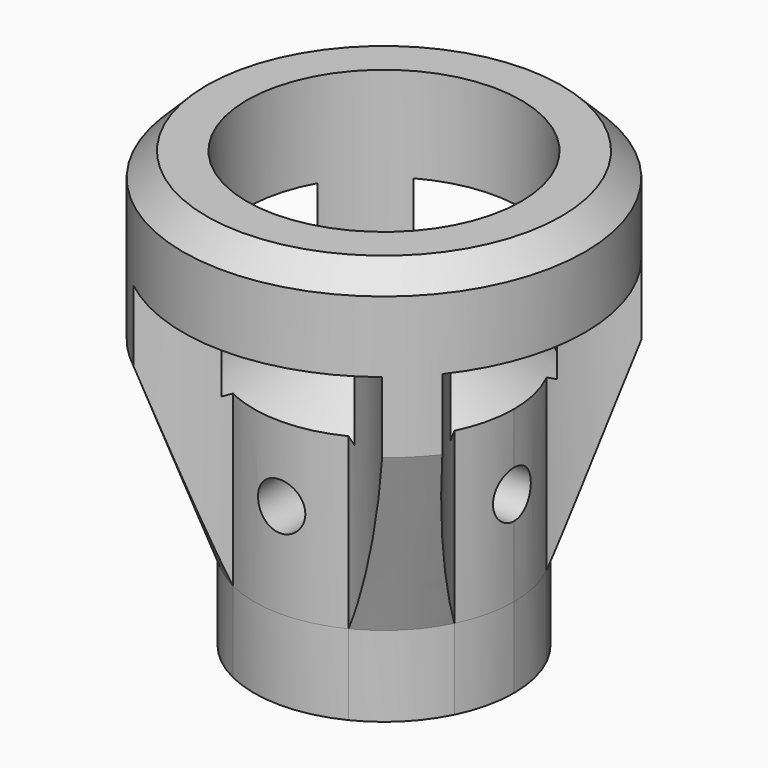
from build123d import *
from build123d import SkipClean  # not in build123d's __all__

# Parameters (mm, degrees)
F2_R          = 0.5
F3_DEPTH      = 4.251
F3_DEPTH_BACK = 4.251
F4_R          = 0.5
F5_DEPTH      = 4.2510001
F5_DEPTH_BACK = 4.2510001
F7_DEPTH      = 7.2
F8_SIZE2      = 0.5
F8_SIZE       = 0.5


with BuildPart() as f1:
    # F0 (on Front) → F1 (revolve)
    with BuildSketch(Plane.XZ):
        Polygon((0.75, 1), (0.75, 0), (2.75, 0), (2.75, 1.7), (4.25, 5.7), (4.25, 9.2), (2.9, 9.2), (2.9, 5.2), (0.75, 6.4413030788), (0.75, 2.7505553499), (0.1, 2.375277675), (0.1, 1.375277675), align=None)
    revolve(axis=Axis((0, 0, 4.6), (0, 0, -1)))

    # F2 (on Front) → F3 (cut, two sides)
    with BuildSketch(Plane.XZ) as f3_sk:
        with Locations((0, 3.7)):
            Circle(F2_R)
    extrude(amount=-F3_DEPTH, mode=Mode.SUBTRACT)
    extrude(f3_sk.sketch, amount=F3_DEPTH_BACK, mode=Mode.SUBTRACT)

    # F4 (on Right) → F5 (cut, two sides)
    with BuildSketch(Plane.YZ) as f5_sk:
        with Locations((0, 3.7)):
            Circle(F4_R)
    extrude(amount=-F5_DEPTH, mode=Mode.SUBTRACT)
    extrude(f5_sk.sketch, amount=F5_DEPTH_BACK, mode=Mode.SUBTRACT)

    # F6 (on Top) → F7 (cut)
    with BuildSketch(Plane.XY):
        with BuildLine():
            ThreePointArc((2.6516504294, 3.3587572106), (3.1943648253, 4.0460926544), (3.5628585232, 4.8405618624))
            ThreePointArc((3.5628585232, 4.8405618624), (1.875, 5.7104618903), (0, 6.0104076401))
            Line((0, 6.0104076401), (2.6516504294, 3.3587572106))
        make_face()
        with BuildLine():
            ThreePointArc((1.2201895167, 2.464475105), (1.9868873303, 2.8300336469), (2.6516504294, 3.3587572106))
            Line((2.6516504294, 3.3587572106), (0, 6.0104076401))
            ThreePointArc((0, 6.0104076401), (-1.875, 5.7104618903), (-3.5628585232, 4.8405618624))
            ThreePointArc((-3.5628585232, 4.8405618624), (-2.6703621866, 3.3776019518), (-1.2201895167, 2.464475105))
            ThreePointArc((-1.2201895167, 2.464475105), (0, 2.75), (1.2201895167, 2.464475105))
        make_face()
        with BuildLine():
            ThreePointArc((-3.5628585232, -4.8405618624), (0, -6.0104076401), (3.5628585232, -4.8405618624))
            ThreePointArc((3.5628585232, -4.8405618624), (2.6703621866, -3.3776019518), (1.2201895167, -2.464475105))
            ThreePointArc((1.2201895167, -2.464475105), (0, -2.75), (-1.2201895167, -2.464475105))
            ThreePointArc((-1.2201895167, -2.464475105), (-2.6703621866, -3.3776019518), (-3.5628585232, -4.8405618624))
        make_face()
        with BuildLine():
            ThreePointArc((-4.8405618624, 3.5628585232), (-6.0104076401, 0), (-4.8405618624, -3.5628585232))
            ThreePointArc((-4.8405618624, -3.5628585232), (-3.3776019518, -2.6703621866), (-2.464475105, -1.2201895167))
            ThreePointArc((-2.464475105, -1.2201895167), (-2.75, 0), (-2.464475105, 1.2201895167))
            ThreePointArc((-2.464475105, 1.2201895167), (-3.3776019518, 2.6703621866), (-4.8405618624, 3.5628585232))
        make_face()
        with BuildLine():
            Line((3.3587572106, 2.6516504294), (6.0104076401, 0))
            ThreePointArc((6.0104076401, 0), (5.7104618903, 1.875), (4.8405618624, 3.5628585232))
            ThreePointArc((4.8405618624, 3.5628585232), (4.0460926544, 3.1943648253), (3.3587572106, 2.6516504294))
        make_face()
        with BuildLine():
            ThreePointArc((4.8405618624, -3.5628585232), (5.7104618903, -1.875), (6.0104076401, 0))
            Line((6.0104076401, 0), (3.3587572106, 2.6516504294))
            ThreePointArc((3.3587572106, 2.6516504294), (2.8300336469, 1.9868873303), (2.464475105, 1.2201895167))
            ThreePointArc((2.464475105, 1.2201895167), (2.6776675054, 0.626575399), (2.75, 0))
            ThreePointArc((2.75, 0), (2.6776675054, -0.626575399), (2.464475105, -1.2201895167))
            ThreePointArc((2.464475105, -1.2201895167), (3.3776019518, -2.6703621866), (4.8405618624, -3.5628585232))
        make_face()
    with SkipClean():  # cleaning this boolean's faces spoils the solid; the shape is the same uncleaned
        extrude(amount=F7_DEPTH, mode=Mode.SUBTRACT)

    # F8
    f8_edges = [f1.edges().sort_by_distance(p)[0] for p in [
        (-4.25, 0, 9.2),
    ]]
    chamfer(f8_edges, length=F8_SIZE, length2=F8_SIZE2)


solid = f1.part
